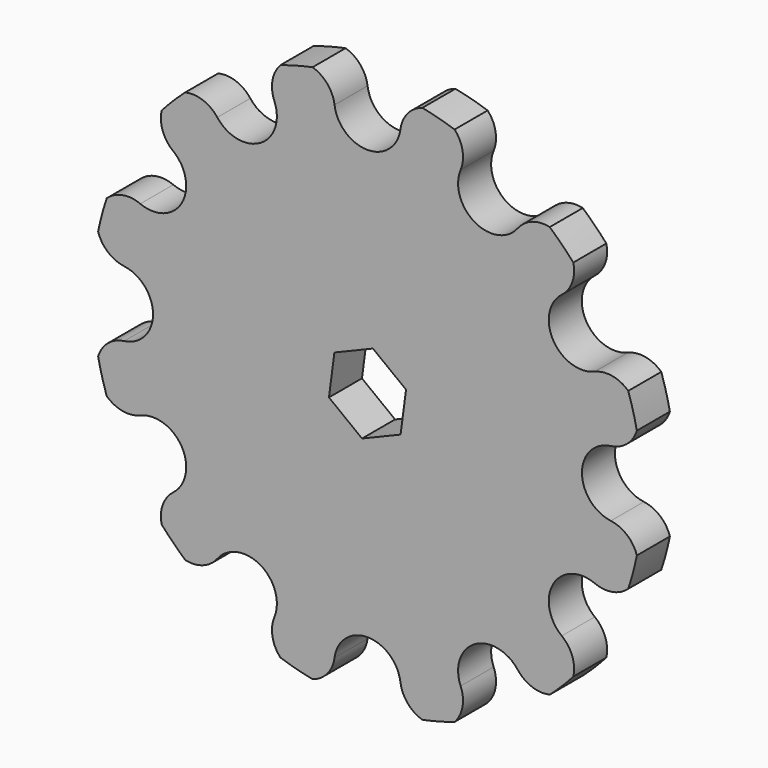
from build123d import *

# Parameters (mm, degrees)
F0_R            = 42.2899684473
F1_DEPTH        = 6.35
F3_DEPTH        = 6.351
F3_COPIES_COUNT = 12
F5_DEPTH        = 6.351


# Not quite as in the source:
# - a pattern or mirror of a feature is missing from the dataset's text; its kind, count and spacing are read off the source's solid


with BuildPart() as f1:
    # F0 (on Front) → F1 (new body)
    with BuildSketch(Plane.XZ):
        Circle(F0_R)
    extrude(amount=-F1_DEPTH)

    # F2 (on face) → F3 (cut, through all)
    with BuildSketch(Plane.XZ):
        with BuildLine():
            ThreePointArc((-41.4371280171, -8.4501983983), (-39.9301176937, -6.1715058408), (-37.4314860419, -5.0668068974))
            ThreePointArc((-37.4314860419, -5.0668068974), (-37.42798385, -5.0663435871), (-37.4244819792, -5.065877856))
            ThreePointArc((-37.4244819792, -5.065877856), (-32.9892827736, 0.0035327048), (-37.4314860419, 5.0668068974))
            ThreePointArc((-37.4314860419, 5.0668068974), (-39.9301176937, 6.1715058408), (-41.4371280171, 8.4501983983))
            ThreePointArc((-41.4371280171, 8.4501983983), (-42.2899684473, 0), (-41.4371280171, -8.4501983983))
        make_face()
    f3 = extrude(amount=-F3_DEPTH, mode=Mode.SUBTRACT)

    # F3_copies: F3 ×12 about axis
    f3_copies_axis = Axis((0, 0, 0), (0, 1, 0))
    for i in range(1, F3_COPIES_COUNT):
        add(f3.rotate(f3_copies_axis, i * 360 / F3_COPIES_COUNT), mode=Mode.SUBTRACT)

    # F4 (on face) → F5 (cut, through all)
    with BuildSketch(Plane.XZ):
        Polygon((0.8374305792, 6.3609167663), (-5.0900002214, 3.9056945387), (-5.9274308006, -2.4552222276), (-0.8374305792, -6.3609167663), (5.0900002214, -3.9056945387), (5.9274308006, 2.4552222276), align=None)
    extrude(amount=-F5_DEPTH, mode=Mode.SUBTRACT)


solid = f1.part
